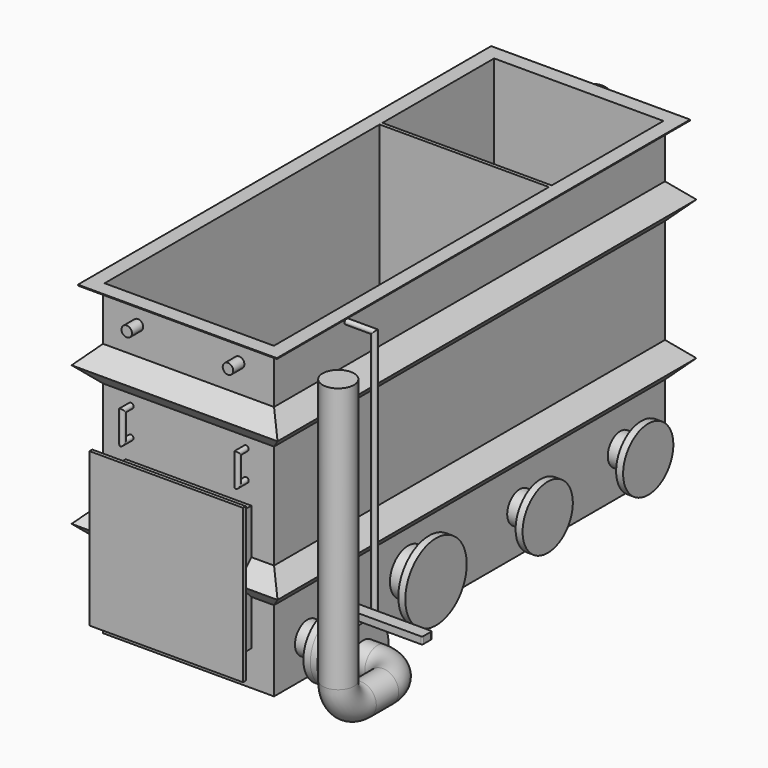
from build123d import *

# Parameters (mm, degrees)
F0_W          = 622.3
F0_H          = 1778
F1_DEPTH      = 558.8
F1_DEPTH_BACK = 558.8
F2_T          = -3.175
F3_W          = 723.9
F3_H          = 1879.6
F3_W_2        = 615.95
F3_H_2        = 1771.65
F4_DEPTH      = 3.175
F7_W          = 457.2
F7_H          = 457.2
F8_DEPTH      = 88.9
F9_W          = 558.8
F9_H          = 558.8
F9_W_2        = 457.2
F9_H_2        = 457.2
F10_DEPTH     = 12.7
F11_R         = 82.55
F11_R_2       = 57.15
F12_DEPTH     = 76.2
F13_R         = 139.7
F13_R_2       = 114.3
F14_DEPTH     = 25.4
F15_R         = 9.525
F18_W         = 615.95
F18_H         = 12.7
F19_DEPTH     = 863.6
F20_R         = 31.75
F21_DEPTH     = 76.2
F22_R         = 12.7
F23_DEPTH     = 50.8
F24_R         = 57.15
F25_DEPTH     = 76.2
F26_R         = 114.3
F27_DEPTH     = 25.4
F28_R         = 114.3
F29_DEPTH     = 25.4
F30_R         = 104.775
F31_DEPTH     = 50.8
F32_R         = 114.3
F33_DEPTH     = 25.4
F34_R         = 57.15
F36_FACE_R    = 57.15
F40_R         = 19.05
F41_DEPTH     = 127
F43_DEPTH     = 25.4
F44_R         = 76.2
F45_DEPTH     = 25.4
F46_R         = 19.05
F47_DEPTH     = 50.8
F48_R         = 9.525


with BuildPart() as f1:
    # F0 (on Top) → F1 (new body, two sides)
    with BuildSketch(Plane.XY) as f1_sk:
        Rectangle(F0_W, F0_H)
    extrude(amount=F1_DEPTH)
    extrude(f1_sk.sketch, amount=-F1_DEPTH_BACK)

    # F2
    f2_openings = [f1.faces().sort_by_distance(p)[0] for p in [
        (0, 0, 558.8),
    ]]
    offset(amount=F2_T, openings=f2_openings)

    # F3 (on face) → F4 (join)
    with BuildSketch(Plane.XY.offset(558.8)):
        Rectangle(F3_W, F3_H)
        Rectangle(F3_W_2, F3_H_2, mode=Mode.SUBTRACT)
    extrude(amount=F4_DEPTH)

    # F6: sweep along a path in F6_path
    with BuildLine(Plane(origin=(-311.15, -889, -558.8), x_dir=(0, -1, 0), z_dir=(0, 0, -1))) as f6_path:
        Line((0, 0), (0, -622.3))
        Line((0, -622.3), (-1778, -622.3))
        Line((-1778, -622.3), (-1778, 0))
        Line((-1778, 0), (0, 0))
    # F5 (on face) → F6 (sweep)
    with BuildSketch(Plane.YZ.offset(311.15)):
        Polygon((-889, 241.3), (-889, 368.3), (-952.5, 304.8), align=None)
        Polygon((-889, -266.7), (-889, -139.7), (-952.5, -203.2), align=None)
    sweep(path=f6_path.line, transition=Transition.RIGHT)

    # F7 (on face) → F8 (join)
    with BuildSketch(Plane.XZ.offset(889)):
        with Locations((0, -203.2)):
            Rectangle(F7_W, F7_H)
    extrude(amount=F8_DEPTH)

    # F9 (on face) → F10 (join)
    with BuildSketch(Plane.XZ.offset(977.9)):
        with Locations((0, -203.2)):
            Rectangle(F9_W, F9_H)
        with Locations((0, -203.2)):
            Rectangle(F9_W_2, F9_H_2, mode=Mode.SUBTRACT)
        with Locations((0, -203.2)):
            Rectangle(F9_W_2, F9_H_2)
    extrude(amount=F10_DEPTH)

    # F11 (on face) → F12 (join)
    with BuildSketch(Plane.YZ.offset(311.15)):
        with Locations((-279.4, -406.4)):
            Circle(F11_R)
        with Locations((228.6, -406.4)):
            Circle(F11_R_2)
        with Locations((685.8, -406.4)):
            Circle(F11_R_2)
    extrude(amount=F12_DEPTH)

    # F13 (on face) → F14 (join)
    with BuildSketch(Plane.YZ.offset(387.35)):
        with Locations((-279.4, -406.4)):
            Circle(F13_R)
        with Locations((228.6, -406.4)):
            Circle(F13_R_2)
        with Locations((685.8, -406.4)):
            Circle(F13_R_2)
    extrude(amount=F14_DEPTH)

    # F17: sweep along a path in F16
    with BuildLine(Plane.XZ.offset(889)) as f17_path:
        Line((311.15, 508), (412.75, 508))
        Line((412.75, 508), (412.75, -508))
        Line((412.75, -508), (311.15, -508))
    # F15 (on face) → F17 (sweep)
    with BuildSketch(Plane.YZ.offset(311.15)):
        with Locations((-558.8, 508)):
            Circle(F15_R)
    sweep(path=f17_path.line, transition=Transition.RIGHT)

    # F18 (on face) → F19 (join)
    with BuildSketch(Plane.XY.offset(561.975)):
        with Locations((0, 371.475)):
            Rectangle(F18_W, F18_H)
    extrude(amount=-F19_DEPTH)

    # F20 (on face) → F21 (join)
    with BuildSketch(Plane(origin=(0, 889, 0), x_dir=(-1, 0, 0), z_dir=(0, 1, 0))):
        with Locations((0, 457.2)):
            Circle(F20_R)
        with Locations((0, -469.9)):
            Circle(F20_R)
    extrude(amount=F21_DEPTH)

    # F22 (on face) → F23 (join)
    with BuildSketch(Plane(origin=(0, 889, 0), x_dir=(-1, 0, 0), z_dir=(0, 1, 0))):
        with Locations((-76.2, -355.6)):
            Circle(F22_R)
    extrude(amount=F23_DEPTH)

    # F24 (on face) → F25 (join)
    with BuildSketch(Plane.YZ.offset(311.15)):
        with Locations((-736.6, -431.8)):
            Circle(F24_R)
    extrude(amount=F25_DEPTH)

    # F26 (on face) → F27 (join)
    with BuildSketch(Plane.YZ.offset(387.35)):
        with Locations((-736.6, -431.8)):
            Circle(F26_R)
    extrude(amount=F27_DEPTH)

    # F44 (on face) → F45 (join)
    with BuildSketch(Plane(origin=(0, 965.2, 0), x_dir=(-1, 0, 0), z_dir=(0, 1, 0))):
        with Locations((0, 457.2)):
            Circle(F44_R)
        with Locations((0, -469.9)):
            Circle(F44_R)
    extrude(amount=F45_DEPTH)

    # F46 (on face) → F47 (join)
    with BuildSketch(Plane.XZ.offset(889)):
        with Locations((-184.15, 469.9)):
            Circle(F46_R)
        with Locations((184.15, 469.9)):
            Circle(F46_R)
    extrude(amount=F47_DEPTH)

    # F50: sweep along a path in F49
    with BuildLine(Plane.YZ.offset(311.15)) as f50_path:
        Line((-889, 215.9), (-939.8, 215.9))
        Line((-939.8, 215.9), (-939.8, 88.9))
        Line((-939.8, 88.9), (-889, 88.9))
    # F48 (on face) → F50 (sweep)
    with BuildSketch(Plane.XZ.offset(889)):
        with Locations((-209.55, 203.2)):
            Circle(F48_R)
        with Locations((209.55, 203.2)):
            Circle(F48_R)
    sweep(path=f50_path.line, transition=Transition.RIGHT)


with BuildPart() as f29:
    # F28 (on face) → F29 (new body)
    with BuildSketch(Plane.YZ.offset(412.75)):
        with Locations((-736.6, -431.8)):
            Circle(F28_R)
    extrude(amount=F29_DEPTH)


with BuildPart() as f31:
    # F30 (on face) → F31 (new body)
    with BuildSketch(Plane.YZ.offset(438.15)):
        with Locations((-736.6, -431.8)):
            Circle(F30_R)
    extrude(amount=F31_DEPTH)

    # F40 (on plane+point) → F41 (join)
    with BuildSketch(Plane(origin=(0, 0, -431.8), x_dir=(1, 0, 0), z_dir=(0, 0, -1))):
        with Locations((463.55, 736.6)):
            Circle(F40_R)
    extrude(amount=-F41_DEPTH)

    # F42 (on face) → F43 (join)
    with BuildSketch(Plane.XY.offset(-304.8)):
        with BuildLine():
            Line((741.045, -714.375), (446.405, -714.375))
            ThreePointArc((446.405, -714.375), (442.8128975516, -715.8628975516), (441.325, -719.455))
            Line((441.325, -719.455), (441.325, -753.745))
            ThreePointArc((441.325, -753.745), (442.8128975516, -757.3371024484), (446.405, -758.825))
            Line((446.405, -758.825), (741.045, -758.825))
            ThreePointArc((741.045, -758.825), (744.6371024484, -757.3371024484), (746.125, -753.745))
            Line((746.125, -753.745), (746.125, -719.455))
            ThreePointArc((746.125, -719.455), (744.6371024484, -715.8628975516), (741.045, -714.375))
        make_face()
    extrude(amount=F43_DEPTH)


with BuildPart() as f33:
    # F32 (on face) → F33 (new body)
    with BuildSketch(Plane.YZ.offset(488.95)):
        with Locations((-736.6, -431.8)):
            Circle(F32_R)
    extrude(amount=F33_DEPTH)


with BuildPart() as f36:
    # F36: sweep along a path in F35
    with BuildLine(Plane(origin=(0, 0, -558.8), x_dir=(1, 0, 0), z_dir=(0, 0, -1))) as f36_path:
        Line((514.35, 736.6), (565.15, 736.6))
        ThreePointArc((565.15, 736.6), (636.9920489686, 766.3579510314), (666.75, 838.2))
        Line((666.75, 838.2), (666.75, 889))
    # F34 (on face) → F36 (sweep)
    with BuildSketch(Plane.YZ.offset(514.35)):
        with Locations((-736.6, -431.8)):
            Circle(F34_R)
    sweep(path=f36_path.line)

    # F38: sweep along a path in F37
    with BuildLine(Plane.YZ.offset(311.15)) as f38_path:
        Line((-889, -431.8), (-939.8, -431.8))
        ThreePointArc((-939.8, -431.8), (-1011.6420489686, -402.0420489686), (-1041.4, -330.2))
        Line((-1041.4, -330.2), (-1041.4, 635))
    # F36_face (on face) → F38 (sweep)
    with BuildSketch(Plane(origin=(666.75, -889, -431.8), x_dir=(1, 0, 0), z_dir=(0, -1, 0))):
        Circle(F36_FACE_R)
    sweep(path=f38_path.line)


solid = Compound([f1.part, f29.part, f31.part, f33.part, f36.part])
